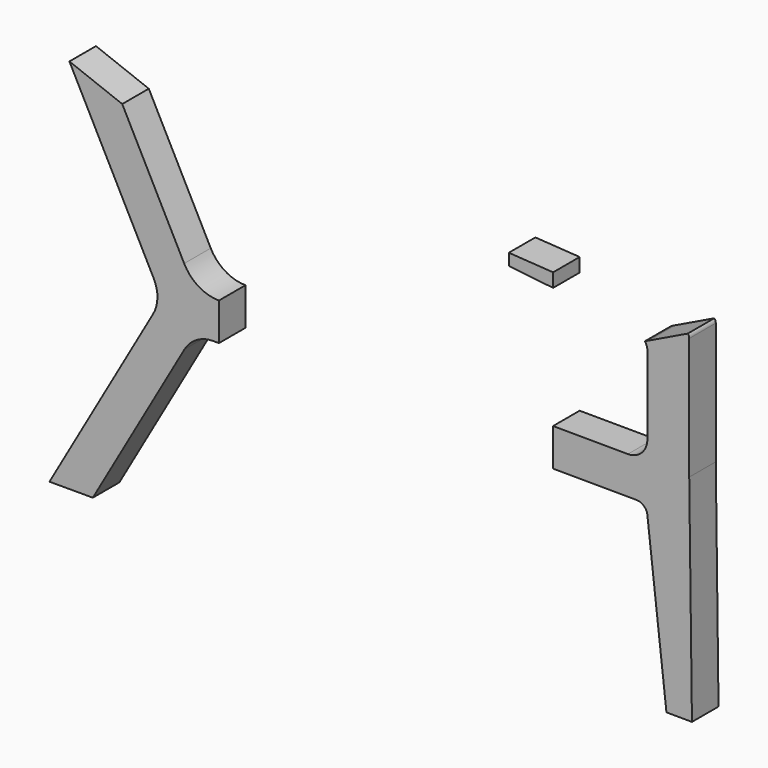
from build123d import *

# Parameters (mm, degrees)
F1_DEPTH = 30


with BuildPart() as f1:
    # F0 (on Front) → F1 (new body, symmetric)
    with BuildSketch(Plane.XZ):
        with BuildLine():
            Line((792.9128824881, 118.9643679948), (787.9878913216, 506.8038779257))
            Line((787.9878913216, 506.8038779257), (787.9878913216, 683.6658184119))
            add(Edge.make_bspline(
                [(714.5339111446, 700.0838076709), (739.5925972645, 695.0095645709), (764.0533999142, 689.5203425349), (787.9878913215, 683.6658184119)],
                knots=[0.5636173816, 0.5636173816, 0.5636173816, 0.5636173816, 0.6158564512, 0.6158564512, 0.6158564512, 0.6158564512], degree=3))
            Line((714.5339111446, 700.0838076709), (707.766144209, 696.8138969939))
            ThreePointArc((707.766144209, 696.8138969939), (711.16675882, 690.8444986797), (712.3467062191, 684.0765137432))
            Line((712.3467062191, 684.0765137432), (712.3467062191, 542.3923685329))
            ThreePointArc((712.3467062191, 542.3923685329), (702.0295939995, 517.5779563734), (677.1607033152, 507.3928627804))
            Line((677.1607033152, 507.3928627804), (541.9986248016, 508.1111740414))
            Line((541.9986248016, 508.1111740414), (541.9986248016, 477.4119283793))
            Line((541.9986248016, 477.4119283793), (541.9986248016, 440.2998282791))
            Line((541.9986248016, 440.2998282791), (692.7038248536, 439.500422329))
            ThreePointArc((692.7038248536, 439.500422329), (706.6874970919, 433.6950222298), (712.5961253131, 419.7546537941))
            Line((712.5961253131, 419.7546537941), (746.8222238447, 119.2088529014))
            Line((746.8222238447, 119.2088529014), (746.9060652922, 119.2084081699))
            Line((746.9060652922, 119.2084081699), (792.9128824881, 118.9643679948))
        make_face()
        with BuildLine():
            add(Edge.make_bspline(
                [(714.5339111446, 700.0838076709), (739.5925972645, 695.0095645709), (764.0533999142, 689.5203425349), (787.9878913215, 683.6658184119)],
                knots=[0.5636173816, 0.5636173816, 0.5636173816, 0.5636173816, 0.6158564512, 0.6158564512, 0.6158564512, 0.6158564512], degree=3))
            Line((787.9878913216, 683.6658184119), (787.9878913216, 727.4259827856))
            ThreePointArc((787.9878913216, 727.4259827856), (787.2869015502, 731.1040813117), (785.2822095679, 734.2665179489))
            Line((785.2822095679, 734.2665179489), (714.5339111446, 700.0838076709))
        make_face()
        Polygon((746.916581268, 118.3802826414), (746.9060652922, 119.2084081699), (746.8222238447, 119.2088529014), align=None)
    extrude(amount=F1_DEPTH, both=True)


with BuildPart() as f1b:
    # F0 (on Front) → F1, piece 2 (new body, symmetric)
    with BuildSketch(Plane.XZ):
        with BuildLine():
            add(Edge.make_bspline(
                [(461.9986116886, 736.7730380501), (489.0719013944, 734.0640894482), (515.7548604152, 731.0842201394), (541.9986248016, 727.7995146356)],
                knots=[0.3993309236, 0.3993309236, 0.3993309236, 0.3993309236, 0.4493215774, 0.4493215774, 0.4493215774, 0.4493215774], degree=3))
            Line((541.9986248016, 727.7995146356), (541.9986248016, 752.614573807))
            Line((541.9986248016, 752.614573807), (461.9986116886, 757.7564887194))
            Line((461.9986116886, 757.7564887194), (461.9986116886, 736.7730380501))
        make_face()
    extrude(amount=F1_DEPTH, both=True)


with BuildPart() as f1c:
    # F0 (on Front) → F1, piece 3 (new body, symmetric)
    with BuildSketch(Plane.XZ):
        with BuildLine():
            Line((-124.6641682472, 549.8122041474), (-236.6087170305, 767.1163282575))
            Line((-236.6087170305, 767.1163282575), (-332.0290716681, 803.8758623378))
            Line((-332.0290716686, 803.8758623375), (-179.5995307623, 507.9832241058))
            ThreePointArc((-179.5995307623, 507.9832241058), (-173.0083340294, 479.445603769), (-180.8329047313, 451.2212217175))
            Line((-180.8329047313, 451.2212217175), (-368.0669905303, 123.5615715693))
            Line((-368.0669905303, 123.5615715693), (-289.7571332166, 123.5615715693))
            Line((-289.7571332166, 123.5615715693), (-124.031344359, 413.5817020702))
            ThreePointArc((-124.031344359, 413.5817020702), (-102.1015120603, 435.6000196795), (-72.0613854071, 443.5570697393))
            Line((-72.0613854071, 443.5570697393), (-61.9120658447, 443.5032333325))
            Line((-61.9120658447, 443.5032333325), (-61.9120658447, 477.4119283793))
            Line((-61.9120658447, 477.4119283793), (-61.9120658447, 511.3206234261))
            ThreePointArc((-61.9120658447, 511.3206234261), (-98.6652755529, 521.8001330848), (-124.6641682472, 549.8122041474))
        make_face()
    extrude(amount=F1_DEPTH, both=True)


solid = Compound([f1.part, f1b.part, f1c.part])
